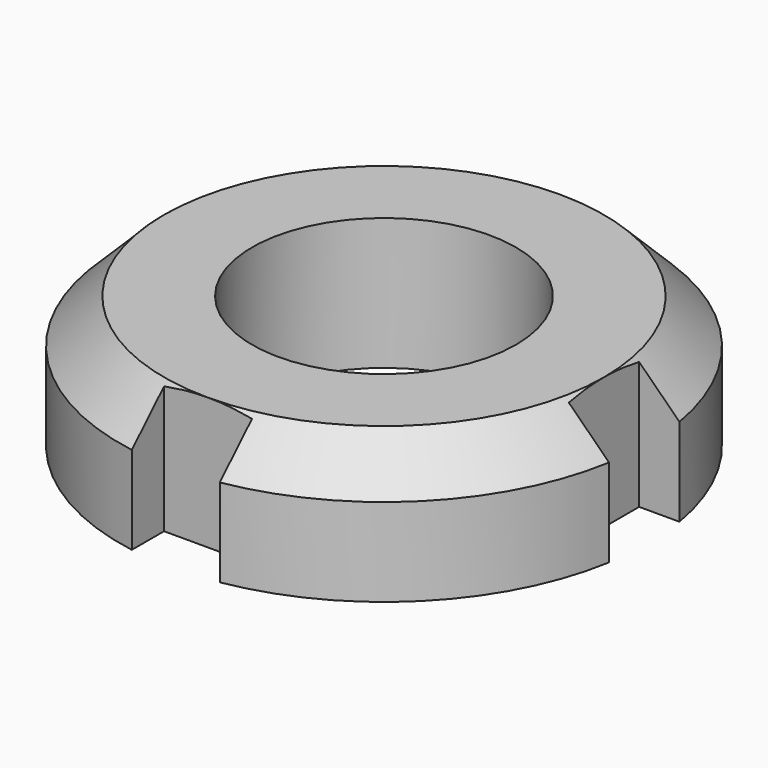
from build123d import *

# Parameters (mm, degrees)
F0_R     = 3
F1_DEPTH = 3
F2_SIZE  = 0.99999


# Not quite as in the source:
# - a fillet or chamfer is up to 0.001 mm smaller than in the source, because OpenCascade refuses the exact size


with BuildPart() as f1:
    # F0 (on Top) → F1 (new body)
    with BuildSketch(Plane.XY):
        with BuildLine():
            Line((-1, 5), (-1, 5.9160797831))
            ThreePointArc((-1, 5.9160797831), (-4.2426406871, 4.2426406871), (-5.9160797831, 1))
            Line((-5.9160797831, 1), (-5, 1))
            Line((-5, 1), (-5, -1))
            Line((-5, -1), (-5.9160797831, -1))
            ThreePointArc((-5.9160797831, -1), (-4.2426406871, -4.2426406871), (-1, -5.9160797831))
            Line((-1, -5.9160797831), (-1, -5))
            Line((-1, -5), (1, -5))
            Line((1, -5), (1, -5.9160797831))
            ThreePointArc((1, -5.9160797831), (4.2426406871, -4.2426406871), (5.9160797831, -1))
            Line((5.9160797831, -1), (5, -1))
            Line((5, -1), (5, 1))
            Line((5, 1), (5.9160797831, 1))
            ThreePointArc((5.9160797831, 1), (4.2426406871, 4.2426406871), (1, 5.9160797831))
            Line((1, 5.9160797831), (1, 5))
            Line((1, 5), (-1, 5))
        make_face()
        Circle(F0_R, mode=Mode.SUBTRACT)
    extrude(amount=F1_DEPTH)

    # F2 (size 1 in the source; OpenCascade refuses exactly that, so slightly less here)
    f2_edges = [f1.edges().sort_by_distance(p)[0] for p in [
        (-4.242641, -4.242641, 3),
        (-4.242641, 4.242641, 3),
        (4.242641, 4.242641, 3),
        (4.242641, -4.242641, 3),
    ]]
    chamfer(f2_edges, length=F2_SIZE)


solid = f1.part
